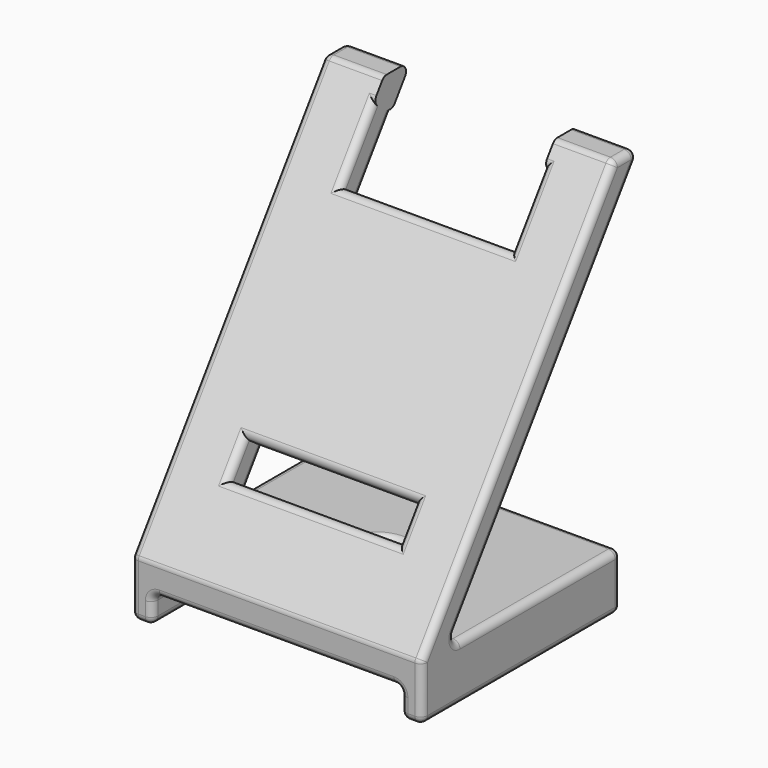
from build123d import *

# Parameters (mm, degrees)
F0_W      = 52.7558
F0_H      = 45.1358
F1_DEPTH  = 5.08
F2_W      = 3.81
F2_H      = 45.1358
F3_DEPTH  = 5.08
F4_R      = 4.953
F5_DEPTH  = 25.4
F7_DEPTH  = 26.3779
F8_W      = 30.988
F8_H      = 12.7
F9_DEPTH  = 46.7108254453
F10_W     = 30.988
F10_H     = 6.35
F11_DEPTH = 5.08
F12_F1_R  = 1.27
F12_F2_R  = 1.27
F13_W     = 30.988
F13_H     = 7.8715959617
F13_H_2   = 2.2884040383
F14_DEPTH = 25.4


with BuildPart() as f1:
    # F0 (on Top) → F1 (new body)
    with BuildSketch(Plane.XY):
        Rectangle(F0_W, F0_H)
    extrude(amount=F1_DEPTH)

    # F2 (on Top) → F3 (join)
    with BuildSketch(Plane.XY):
        with Locations((24.4729, 0)):
            Rectangle(F2_W, F2_H)
        with Locations((-24.4729, 0)):
            Rectangle(F2_W, F2_H)
    extrude(amount=-F3_DEPTH)

    # F4 (on Top) → F5 (cut)
    with BuildSketch(Plane.XY):
        Circle(F4_R)
    extrude(amount=F5_DEPTH, mode=Mode.SUBTRACT)

    # F6 (on Right) → F7 (join, symmetric)
    with BuildSketch(Plane.YZ):
        Polygon((21.1386244499, 67.4993857748), (-22.5679, 5.08), (-16.3663650891, 5.08), (27.3401593609, 67.4993857748), align=None)
    extrude(amount=F7_DEPTH, both=True)

    # F8 (on face) → F9 (cut, through all)
    with BuildSketch(Plane(origin=(0, -17.5301074531, 12.2747133843), x_dir=(1, 0, 0), z_dir=(0, -0.8191520443, 0.5735764364))):
        with Locations((0, 56.8473525345)):
            Rectangle(F8_W, F8_H)
    extrude(amount=-F9_DEPTH, mode=Mode.SUBTRACT)

    # F10 (on face) → F11 (cut, through all)
    with BuildSketch(Plane(origin=(0, -17.5301074531, 12.2747133843), x_dir=(1, 0, 0), z_dir=(0, -0.8191520443, 0.5735764364))):
        with Locations((0, 9.2223525345)):
            Rectangle(F10_W, F10_H)
    extrude(amount=-F11_DEPTH, mode=Mode.SUBTRACT)

    # F12: fillet of radius 1.27 on 49 edges, made by hand

    # F12_f1
    f12_f1_edges = [f1.edges().sort_by_distance(p)[0] for p in [
        (0, -16.3663650891, 5.08),
        (22.5679, 0, 0),
        (-22.5679, 0, 0),
    ]]
    fillet(f12_f1_edges, radius=F12_F1_R)

    # F12_f2
    f12_f2_edges = [f1.edges().sort_by_distance(p)[0] for p in [
        (26.3779, 4.3205911061, 5.08),
        (26.3779, 22.5679, 0),
        (26.3779, 0, -5.08),
        (26.3779, -22.5679, 0),
        (26.3779, -0.714637775, 36.2896928874),
        (26.3779, 24.2393919054, 67.4993857748),
        (26.3779, 6.1865592384, 37.2889139245),
        (-26.3779, 22.5679, 0),
        (-26.3779, 4.3205911061, 5.08),
        (-26.3779, 6.1865592384, 37.2889139245),
        (-26.3779, 24.2393919054, 67.4993857748),
        (-26.3779, -0.714637775, 36.2896928874),
        (-26.3779, -22.5679, 0),
        (-26.3779, 0, -5.08),
        (0, 21.1386244499, 67.4993857748),
        (0, -22.5679, 5.08),
        (0, 11.4339840588, 53.6397229441),
        (-15.494, 15.0761944297, 58.8413384253),
        (15.494, 15.0761944297, 58.8413384253),
        (0, 18.7184048005, 64.0429539066),
        (0, -14.061488537, 17.2284145755),
        (15.494, -12.2403833515, 19.8292223161),
        (0, -10.4192781661, 22.4300300567),
        (-15.494, -12.2403833515, 19.8292223161),
        (0, 27.3401593609, 67.4993857748),
        (-15.494, -8.0790909666, 16.9154540194),
        (0, -6.2579857811, 19.51626176),
        (15.494, -8.0790909666, 16.9154540194),
        (0, -9.900196152, 14.3146462788),
        (0, 15.5952764438, 50.7259546475),
        (15.494, 19.2374868147, 55.9275701287),
        (-15.494, 19.2374868147, 55.9275701287),
        (0, 22.8796971855, 61.1291856099),
        (0, 22.5679, 5.08),
        (-4.953, 0, 5.08),
        (-24.4729, 22.5679, -5.08),
        (-22.5679, 22.5679, -3.175),
        (0, 22.5679, 0),
        (22.5679, 22.5679, -3.175),
        (24.4729, 22.5679, -5.08),
        (-22.5679, -22.5679, -3.175),
        (-22.5679, 0, -5.08),
        (24.4729, -22.5679, -5.08),
        (22.5679, 0, -5.08),
        (-24.4729, -22.5679, -5.08),
        (0, -22.5679, 0),
        (-22.1959256121, -22.5679, -0.3719743879),
        (22.1959256121, -22.5679, -0.3719743879),
        (22.1959256121, 22.5679, -0.3719743879),
        (-22.1959256121, 22.5679, -0.3719743879),
        (-26.3779, -15.053221546, 5.7635792612),
        (26.3779, -15.053221546, 5.7635792612),
    ]]
    fillet(f12_f2_edges, radius=F12_F2_R)

    # F13 (on face) → F14 (cut)
    with BuildSketch(Plane(origin=(0, -17.5301074531, 12.2747133843), x_dir=(1, 0, 0), z_dir=(0, -0.8191520443, 0.5735764364))):
        with Locations((0, 70.6915545537)):
            Rectangle(F13_W, F13_H)
        with Locations((0, 65.6115545537)):
            Rectangle(F13_W, F13_H_2)
        Polygon((-15.494, 63.4007958817), (-15.494, 56.8473525345), (15.494, 56.8473525345), (15.494, 64.4673525345), (-15.494, 64.4673525345), align=None)
    extrude(amount=-F14_DEPTH, mode=Mode.SUBTRACT)


solid = f1.part
